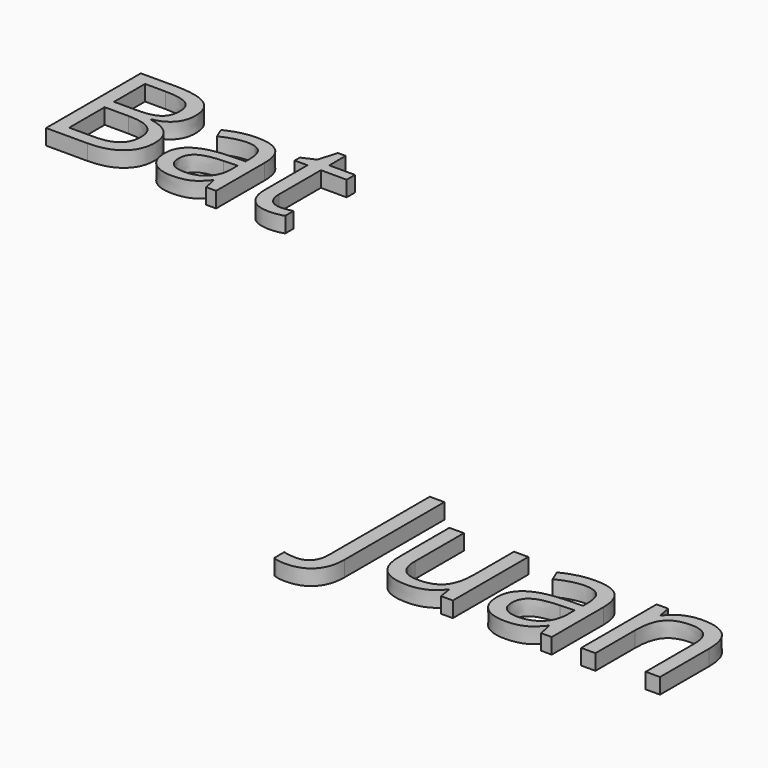
from build123d import *

# Parameters (mm, degrees)
F1_TEXT_SIZE = 14.39333169
F0_TEXT_SIZE = 13.5466663374
F2_DEPTH     = 1.27


# Not quite as in the source:
# - Text() gives the source's letters only with a copy of the font that has no kerning and outlines rounded to 1/6400 em; it was checked with that copy


with BuildPart() as f2:
    # F1 (on Top) + F0 (on Top) → F2 (new body)
    with BuildSketch(Plane.XY):
        with Locations((-24.8412014917, 31.6992066801)):
            Text('Juan', F1_TEXT_SIZE, font='Open Sans', text_align=(TextAlign.LEFT, TextAlign.BOTTOM))
    with BuildSketch(Plane.XY):
        with Locations((-75.742803514, 66.4464011788)):
            Text('Bat', F0_TEXT_SIZE, font='Open Sans', text_align=(TextAlign.LEFT, TextAlign.BOTTOM))
    extrude(amount=F2_DEPTH)


solid = f2.part
